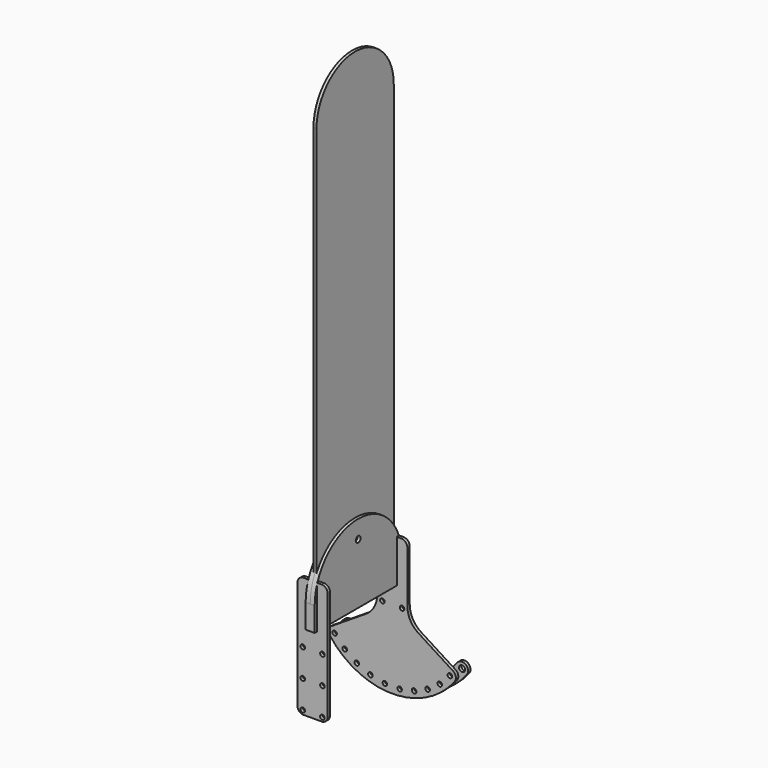
from build123d import *

# Parameters (mm, degrees)
F2_R      = 3.175
F6_DEPTH  = 4.7625
F7_DEPTH  = 1.5875
F3_R      = 2.38125
F8_DEPTH  = 3.175
F4_R      = 2.38125
F9_DEPTH  = 3.175
F5_R      = 3.175
F10_DEPTH = 3.175
F12_DEPTH = 1.5875


# Not quite as in the source:
# - a length typed as a fraction of an inch, garbled in the dataset ("3 / 203.2 mm" for 3/8 in), is restored
# - a feature names something its author has since deleted; it is built from what else it names


with BuildPart() as f6:
    # F2 (on Right) → F6 (new body, symmetric)
    with BuildSketch(Plane.YZ):
        with BuildLine():
            Line((-107.95, 44.45), (-107.95, 19.05))
            Line((-107.95, 19.05), (6.35, 19.05))
            Line((6.35, 19.05), (6.35, 44.45))
            ThreePointArc((6.35, 44.45), (4.7398167984, 57.9203841816), (0, 70.6317207227))
            Line((0, 70.6317207227), (0, 25.4))
            Line((0, 25.4), (-101.6, 25.4))
            Line((-101.6, 25.4), (-101.6, 70.6317207227))
            ThreePointArc((-101.6, 70.6317207227), (-106.3398167984, 57.9203841816), (-107.95, 44.45))
        make_face()
        with BuildLine():
            ThreePointArc((0, 70.6317207227), (-50.8, 101.6), (-101.6, 70.6317207227))
            Line((-101.6, 70.6317207227), (-101.6, 25.4))
            Line((-101.6, 25.4), (0, 25.4))
            Line((0, 25.4), (0, 70.6317207227))
        make_face()
        with Locations((-50.8, 82.55)):
            Circle(F2_R, mode=Mode.SUBTRACT)
    extrude(amount=F6_DEPTH, both=True)

    # F2 (on Right) → F7 (cut, symmetric)
    with BuildSketch(Plane.YZ):
        with BuildLine():
            ThreePointArc((0, 70.6317207227), (-50.8, 101.6), (-101.6, 70.6317207227))
            Line((-101.6, 70.6317207227), (-101.6, 25.4))
            Line((-101.6, 25.4), (0, 25.4))
            Line((0, 25.4), (0, 70.6317207227))
        make_face()
        with Locations((-50.8, 82.55)):
            Circle(F2_R, mode=Mode.SUBTRACT)
    extrude(amount=F7_DEPTH, both=True, mode=Mode.SUBTRACT)


with BuildPart() as f8:
    # F3 (on offset) → F8 (new body)
    with BuildSketch(Plane.XZ.offset(101.6)):
        with BuildLine():
            Line((-4.7625, 64.2817207227), (-9.525, 64.2817207227))
            ThreePointArc((-9.525, 64.2817207227), (-14.0151280605, 62.4218487832), (-15.875, 57.9317207227))
            Line((-15.875, 57.9317207227), (-15.875, -56.3682792773))
            ThreePointArc((-15.875, -56.3682792773), (-14.0151280605, -60.8584073379), (-9.525, -62.7182792773))
            Line((-9.525, -62.7182792773), (9.525, -62.7182792773))
            ThreePointArc((9.525, -62.7182792773), (14.0151280605, -60.8584073379), (15.875, -56.3682792773))
            Line((15.875, -56.3682792773), (15.875, 57.9317207227))
            ThreePointArc((15.875, 57.9317207227), (14.0151280605, 62.4218487832), (9.525, 64.2817207227))
            Line((9.525, 64.2817207227), (4.7625, 64.2817207227))
            Line((4.7625, 64.2817207227), (4.7625, 19.05))
            Line((4.7625, 19.05), (-4.7625, 19.05))
            Line((-4.7625, 19.05), (-4.7625, 64.2817207227))
        make_face()
        with Locations((-10.31875, -58.42)):
            Circle(F3_R, mode=Mode.SUBTRACT)
        with Locations((-10.31875, -29.21)):
            Circle(F3_R, mode=Mode.SUBTRACT)
        with Locations((-10.31875, 0)):
            Circle(F3_R, mode=Mode.SUBTRACT)
        with Locations((10.31875, -58.42)):
            Circle(F3_R, mode=Mode.SUBTRACT)
        with Locations((10.31875, -29.21)):
            Circle(F3_R, mode=Mode.SUBTRACT)
        with Locations((10.31875, 0)):
            Circle(F3_R, mode=Mode.SUBTRACT)
    extrude(amount=F8_DEPTH)


with BuildPart() as f9:
    # F4 (on Front) → F9 (new body)
    with BuildSketch(Plane.XZ):
        with BuildLine():
            Line((4.7625, 19.05), (-4.7625, 19.05))
            Line((-4.7625, 19.05), (-4.7625, 64.2817207227))
            Line((-4.7625, 64.2817207227), (-9.525, 64.2817207227))
            ThreePointArc((-9.525, 64.2817207227), (-14.0151280605, 62.4218487832), (-15.875, 57.9317207227))
            Line((-15.875, 57.9317207227), (-15.875, 3.82142679))
            ThreePointArc((-15.875, 3.82142679), (-19.006140405, -8.3956879406), (-27.627589948, -17.6007159336))
            Line((-27.627589948, -17.6007159336), (-64.0428920913, -40.7998219675))
            ThreePointArc((-64.0428920913, -40.7998219675), (-66.8824421859, -45.0406983115), (-65.6836262099, -50.0016374524))
            ThreePointArc((-65.6836262099, -50.0016374524), (0, -82.55), (65.6836262099, -50.0016374524))
            ThreePointArc((65.6836262099, -50.0016374524), (66.8824421859, -45.0406983115), (64.0428920913, -40.7998219675))
            Line((64.0428920913, -40.7998219675), (27.627589948, -17.6007159336))
            ThreePointArc((27.627589948, -17.6007159336), (19.006140405, -8.3956879406), (15.875, 3.82142679))
            Line((15.875, 3.82142679), (15.875, 57.9317207227))
            ThreePointArc((15.875, 57.9317207227), (14.0151280605, 62.4218487832), (9.525, 64.2817207227))
            Line((9.525, 64.2817207227), (4.7625, 64.2817207227))
            Line((4.7625, 64.2817207227), (4.7625, 19.05))
        make_face()
        with Locations((-37.2452482367, -66.3651854355)):
            Circle(F4_R, mode=Mode.SUBTRACT)
        with Locations((-60.6310395783, -46.1553576484)):
            Circle(F4_R, mode=Mode.SUBTRACT)
        with Locations((-49.9705034386, -57.4548658175)):
            Circle(F4_R, mode=Mode.SUBTRACT)
        with Locations((-22.9810656932, -72.5181531761)):
            Circle(F4_R, mode=Mode.SUBTRACT)
        with Locations((-7.767334093, -75.6595360637)):
            Circle(F4_R, mode=Mode.SUBTRACT)
        with Locations((7.767334093, -75.6595360637)):
            Circle(F4_R, mode=Mode.SUBTRACT)
        with Locations((22.9810656932, -72.5181531761)):
            Circle(F4_R, mode=Mode.SUBTRACT)
        with Locations((37.2452482367, -66.3651854355)):
            Circle(F4_R, mode=Mode.SUBTRACT)
        with Locations((49.9705034386, -57.4548658175)):
            Circle(F4_R, mode=Mode.SUBTRACT)
        with Locations((60.6310395783, -46.1553576484)):
            Circle(F4_R, mode=Mode.SUBTRACT)
        with Locations((-10.31875, 0)):
            Circle(F4_R, mode=Mode.SUBTRACT)
        with Locations((10.31875, 0)):
            Circle(F4_R, mode=Mode.SUBTRACT)
    extrude(amount=-F9_DEPTH)


with BuildPart() as f10:
    # F5 (on offset) → F10 (new body)
    with BuildSketch(Plane.XZ.offset(-19.05)):
        with BuildLine():
            ThreePointArc((-55.1108494471, -42.4492432133), (-64.0170127547, -41.2980459505), (-65.1682100175, -50.2042092581))
            ThreePointArc((-65.1682100175, -50.2042092581), (0.398951337, -82.3467012608), (65.8140635748, -49.8958841502))
            ThreePointArc((65.8140635748, -49.8958841502), (64.6209500594, -40.9952392219), (55.7203051311, -42.1883527374))
            ThreePointArc((55.7203051311, -42.1883527374), (0.3690563144, -69.6467364464), (-55.1108494471, -42.4492432133))
        make_face()
        with Locations((-22.5380164103, -72.5238979115)):
            Circle(F5_R, mode=Mode.SUBTRACT)
        with Locations((-7.361496499, -75.6203674646)):
            Circle(F5_R, mode=Mode.SUBTRACT)
        with Locations((-36.7748383006, -66.4224404811)):
            Circle(F5_R, mode=Mode.SUBTRACT)
        with Locations((8.127646503, -75.5839068692)):
            Circle(F5_R, mode=Mode.SUBTRACT)
        with Locations((23.2894204681, -72.4160226316)):
            Circle(F5_R, mode=Mode.SUBTRACT)
        with Locations((37.4973597502, -66.2476077893)):
            Circle(F5_R, mode=Mode.SUBTRACT)
        with Locations((-49.4837143934, -57.5680998072)):
            Circle(F5_R, mode=Mode.SUBTRACT)
        with Locations((-60.1395297323, -46.3267262357)):
            Circle(F5_R, mode=Mode.SUBTRACT)
        with Locations((50.1644099662, -57.3335335728)):
            Circle(F5_R, mode=Mode.SUBTRACT)
        with Locations((60.767184353, -46.0421184438)):
            Circle(F5_R, mode=Mode.SUBTRACT)
    extrude(amount=F10_DEPTH)


with BuildPart() as f12:
    # F11 (on Right) → F12 (new body, symmetric)
    with BuildSketch(Plane.YZ):
        with BuildLine():
            Line((-101.6, 482.6), (-101.6, 25.4))
            Line((-101.6, 25.4), (-57.15, 25.4))
            Line((-57.15, 25.4), (-57.15, 82.55))
            ThreePointArc((-57.15, 82.55), (-50.8, 88.9), (-44.45, 82.55))
            Line((-44.45, 82.55), (-44.45, 25.4))
            Line((-44.45, 25.4), (0, 25.4))
            Line((0, 25.4), (0, 482.6))
            ThreePointArc((0, 482.6), (-50.8, 533.4), (-101.6, 482.6))
        make_face()
    extrude(amount=F12_DEPTH, both=True)


solid = Compound([f6.part, f8.part, f9.part, f10.part, f12.part])
